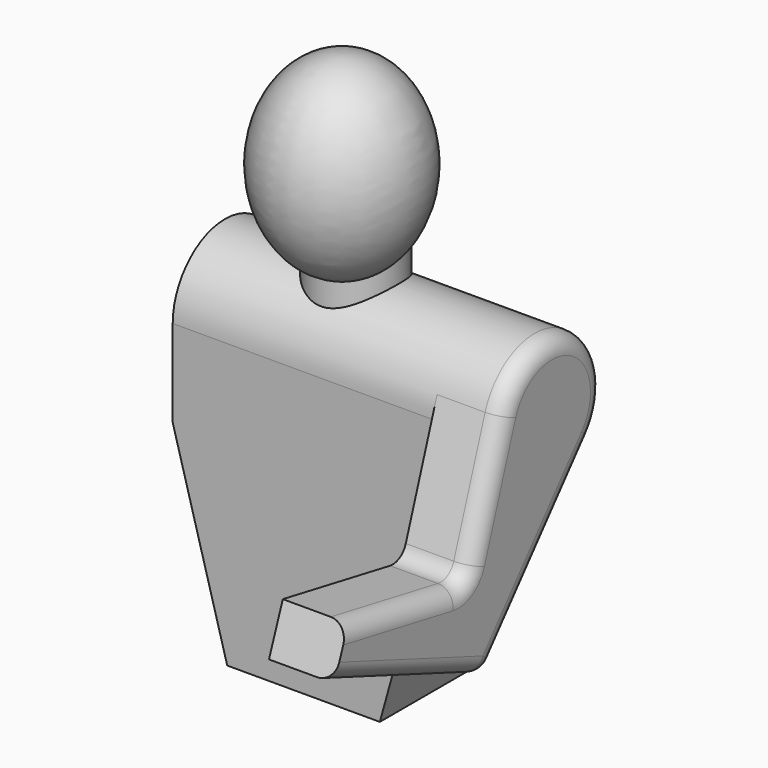
from build123d import *

# Parameters (mm, degrees)
F1_DEPTH    = 19.05
F2_T1_DEPTH = 171.45
F3_W        = 12.7
F3_H        = 38.1
F8_DEPTH    = 19.05
F9_R        = 5.08
F10_R       = 5.08
F11_R       = 5.08


# Not quite as in the source:
# - a fillet or chamfer that OpenCascade refuses, or shapes differently, is made with other operations: its cross-section is extruded or revolved along the edge and cut away or added


with BuildPart() as f1:
    # F0 (on Front) → F1 (new body, symmetric)
    with BuildSketch(Plane.XZ):
        Polygon((-38.1, 57.15), (-22.225, 0), (22.225, 0), (38.1, 57.15), (38.1, 101.6), (-38.1, 101.6), align=None)
    extrude(amount=F1_DEPTH, both=True)

    # F2: fillet of radius 19.05 on 2 edges, made by hand

    # F2_s2 → F2_t1 (cut)
    with BuildSketch(Plane.YZ.offset(-85.725)):
        with BuildLine():
            ThreePointArc((0, 101.6), (-13.4703841816, 96.0203841816), (-19.05, 82.55))
            Line((-19.05, 82.55), (-19.05, 101.6))
            Line((-19.05, 101.6), (0, 101.6))
        make_face()
        with BuildLine():
            ThreePointArc((0, 101.6), (13.4703841816, 96.0203841816), (19.05, 82.55))
            Line((19.05, 82.55), (19.05, 101.6))
            Line((19.05, 101.6), (0, 101.6))
        make_face()
    extrude(amount=F2_T1_DEPTH, mode=Mode.SUBTRACT)

    # F3 (on Front) → F4 (revolve)
    with BuildSketch(Plane.XZ):
        with Locations((6.35, 101.6)):
            Rectangle(F3_W, F3_H)
    revolve(axis=Axis((0, 0, 41.275), (0, 0, -1)))

    # F5 (on Right) → F6 (revolve)
    with BuildSketch(Plane.YZ):
        with BuildLine():
            Line((-5.08, 158.115), (-5.08, 102.235))
            add(Edge.make_bspline(
                [(-5.08, 102.235), (17.145, 102.235), (17.145, 130.175), (17.145, 158.115), (-5.08, 158.115)],
                knots=[3.1415926536, 3.1415926536, 3.1415926536, 4.7123889804, 4.7123889804, 6.2831853072, 6.2831853072, 6.2831853072], degree=2, weights=[1, 0.7071067812, 1, 0.7071067812, 1]))
        make_face()
    revolve(axis=Axis((0, -5.08, 55.275326029), (0, 0, -1)))

    # F7 (on face) → F8 (join)
    with BuildSketch(Plane.YZ.offset(38.1)):
        with BuildLine():
            Line((-23.622, 24.761857734), (14.5931466414, 70.3048960355))
            ThreePointArc((14.5931466414, 70.3048960355), (9.3486979196, 99.1483236264), (-18.0359002739, 88.6826015123))
            Line((-18.0359002739, 88.6826015123), (-30.8627206832, 50.9590916336))
            Line((-30.8627206832, 50.9590916336), (-74.213960244, 59.0636453196))
            Line((-74.213960244, 59.0636453196), (-79.2495722325, 45.6589880743))
            Line((-79.2495722325, 45.6589880743), (-23.622, 24.761857734))
        make_face()
    extrude(amount=F8_DEPTH)

    # F9
    f9_edges = [f1.edges().sort_by_distance(p)[0] for p in [
        (47.625, -30.862721, 50.959092),
    ]]
    fillet(f9_edges, radius=F9_R)

    # F10
    f10_edges = [f1.edges().sort_by_distance(p)[0] for p in [
        (47.625, -23.622, 24.761858),
    ]]
    fillet(f10_edges, radius=F10_R)

    # F11
    f11_edges = [f1.edges().sort_by_distance(p)[0] for p in [
        (57.15, -3.358654, 48.910773),
        (57.15, -53.118999, 35.842741),
        (57.15, -23.91241, 25.868412),
        (57.15, -54.701473, 55.415768),
        (57.15, -31.691239, 52.376034),
        (57.15, -23.740888, 71.904309),
        (57.15, 9.348698, 99.148324),
    ]]
    fillet(f11_edges, radius=F11_R)


solid = f1.part
